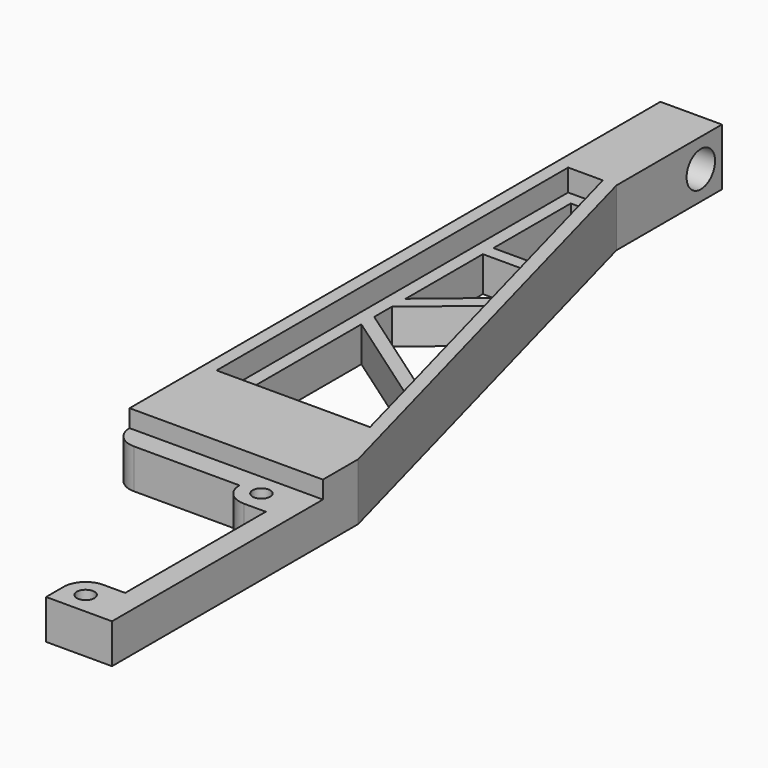
from build123d import *

# Parameters (mm, degrees)
F0_R      = 2
F1_DEPTH  = 9
F2_DEPTH  = 13
F4_DEPTH  = 5
F6_DEPTH  = 8.001
F7_R      = 4.99999
F8_R      = 5
F9_R      = 5
F10_R     = 4.05
F11_DEPTH = 14.001


# Not quite as in the source:
# - a fillet or chamfer is up to 0.001 mm smaller than in the source, because OpenCascade refuses the exact size


with BuildPart() as f1:
    # F0 (on Top) → F1 (new body)
    with BuildSketch(Plane.XY):
        Polygon((8.7753673922, -59.6295086741), (-35.2246326078, -59.6295086741), (-35.2246326078, -64.6295086741), (-6.2246326078, -64.6295086741), (-6.2246326078, -69.6295086741), (3.7753673922, -69.6295086741), (3.7753673922, -109.6295086741), (-6.2246326078, -109.6295086741), (-6.2246326078, -119.6295086741), (8.7753673922, -119.6295086741), align=None)
        with Locations((-1.2246326078, -114.6295086741)):
            Circle(F0_R, mode=Mode.SUBTRACT)
        with Locations((-1.2246326078, -64.6295086741)):
            Circle(F0_R, mode=Mode.SUBTRACT)
    extrude(amount=F1_DEPTH)

    # F0 (on Top) → F2 (join)
    with BuildSketch(Plane.XY):
        Polygon((-21.2246326078, 61.3704913259), (-21.2246326078, 91.3704913259), (-35.2246326078, 91.3704913259), (-35.2246326078, -59.6295086741), (8.7753673922, -59.6295086741), (8.7753673922, -49.6295086741), align=None)
    extrude(amount=F2_DEPTH)

    # F3 (on face) → F4 (cut)
    with BuildSketch(Plane.XY.offset(13)):
        Polygon((2.6947563819, -38.6295086741), (-24.3322706451, 61.3704913259), (-32.2246326078, 61.3704913259), (-32.2246326078, -38.6295086741), align=None)
    extrude(amount=-F4_DEPTH, mode=Mode.SUBTRACT)

    # F5 (on face) → F6 (cut, through all)
    with BuildSketch(Plane.XY.offset(8)):
        Polygon((-26.6290978716, 58.3704913259), (-29.2246326078, 58.3704913259), (-29.2246326078, 36.3704913259), (-20.6831519256, 36.3704913259), align=None)
        Polygon((-19.8723411148, 33.3704913259), (-29.2246326078, 33.3704913259), (-29.2246326078, 11.3704913259), (-16.7414328131, 21.7861306095), align=None)
        Polygon((-15.879765316, 18.5979608701), (-29.2246326078, 7.463369877), (-29.2246326078, 2.463369877), (-7.3999758243, -12.777260249), align=None)
        Polygon((-6.1809639439, -17.2876042066), (-29.2246326078, -1.1957117047), (-29.2246326078, -35.6295086741), (-1.2236924662, -35.6295086741), align=None)
    extrude(amount=-F6_DEPTH, mode=Mode.SUBTRACT)

    # F7 (radius 5 in the source; OpenCascade refuses exactly that, so slightly less here)
    f7_edges = [f1.edges().sort_by_distance(p)[0] for p in [
        (-6.224633, -69.629509, 4.5),
    ]]
    fillet(f7_edges, radius=F7_R)

    # F8
    f8_edges = [f1.edges().sort_by_distance(p)[0] for p in [
        (-6.224633, -109.629509, 4.5),
    ]]
    fillet(f8_edges, radius=F8_R)

    # F9
    f9_edges = [f1.edges().sort_by_distance(p)[0] for p in [
        (-35.224633, -64.629509, 4.5),
    ]]
    fillet(f9_edges, radius=F9_R)

    # F10 (on face) → F11 (cut, through all)
    with BuildSketch(Plane.YZ.offset(-21.2246326078)):
        with Locations((85.3704913259, 6.5)):
            Circle(F10_R)
    extrude(amount=-F11_DEPTH, mode=Mode.SUBTRACT)


solid = f1.part
